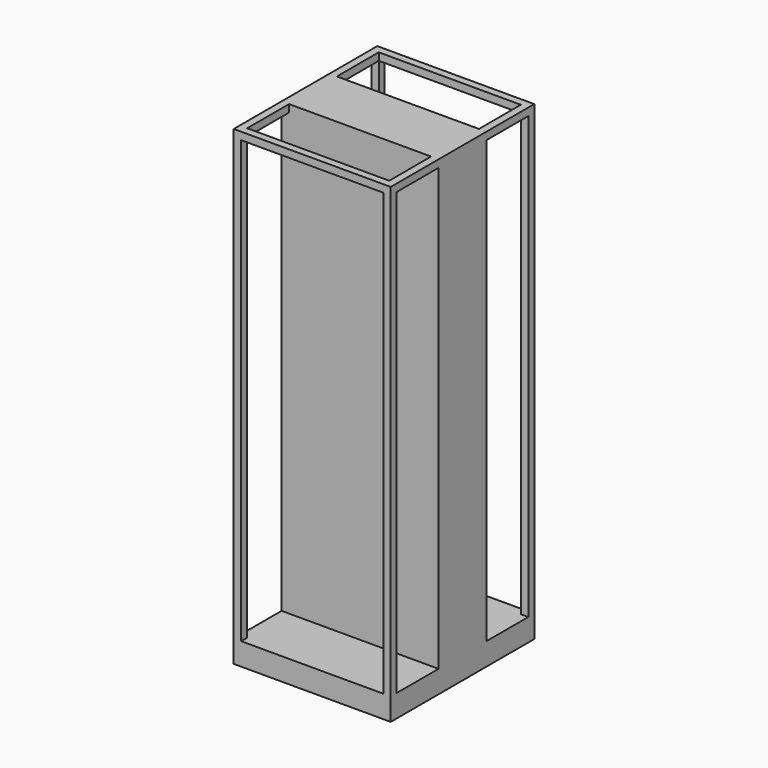
from build123d import *

# Parameters (mm, degrees)
F0_W     = 533.4
F0_H     = 203.2
F1_DEPTH = 1600.2
F2_W     = 177.8
F2_H     = 1498.6
F3_DEPTH = 533.401
F4_W     = 482.6
F4_H     = 177.8
F5_DEPTH = 76.2
F6_W     = 482.6
F6_H     = 1498.6
F7_DEPTH = 50.8


# Not quite as in the source:
# - a pattern or mirror of a feature is missing from the dataset's text; its kind, count and spacing are read off the source's solid


with BuildPart() as f1:
    # F0 (on Top) → F1 (new body)
    with BuildSketch(Plane.XY):
        with Locations((266.7, 508)):
            Rectangle(F0_W, F0_H)
        with Locations((266.7, 101.6)):
            Rectangle(F0_W, F0_H)
        with Locations((266.7, 304.8)):
            Rectangle(F0_W, F0_H)
    extrude(amount=F1_DEPTH)

    # F2 (on face) → F3 (cut, through all)
    with BuildSketch(Plane(origin=(0, 0, 0), x_dir=(0, -1, 0), z_dir=(-1, 0, 0))):
        with Locations((-495.3, 825.5)):
            Rectangle(F2_W, F2_H)
        with Locations((-114.3, 825.5)):
            Rectangle(F2_W, F2_H)
    extrude(amount=-F3_DEPTH, mode=Mode.SUBTRACT)

    # F4 (on face) → F5 (cut)
    with BuildSketch(Plane.XY.offset(1600.2)):
        with Locations((266.7, 495.3)):
            Rectangle(F4_W, F4_H)
        with Locations((266.7, 114.3)):
            Rectangle(F4_W, F4_H)
    extrude(amount=-F5_DEPTH, mode=Mode.SUBTRACT)

    # F6 (on face) → F7 (cut)
    with BuildSketch(Plane.XZ):
        with Locations((266.7, 825.5)):
            Rectangle(F6_W, F6_H)
    f7 = extrude(amount=-F7_DEPTH, mode=Mode.SUBTRACT)

    # F7_copies: F7 across plane
    add(f7.mirror(Plane.ZX.offset(304.8)), mode=Mode.SUBTRACT)


solid = f1.part
